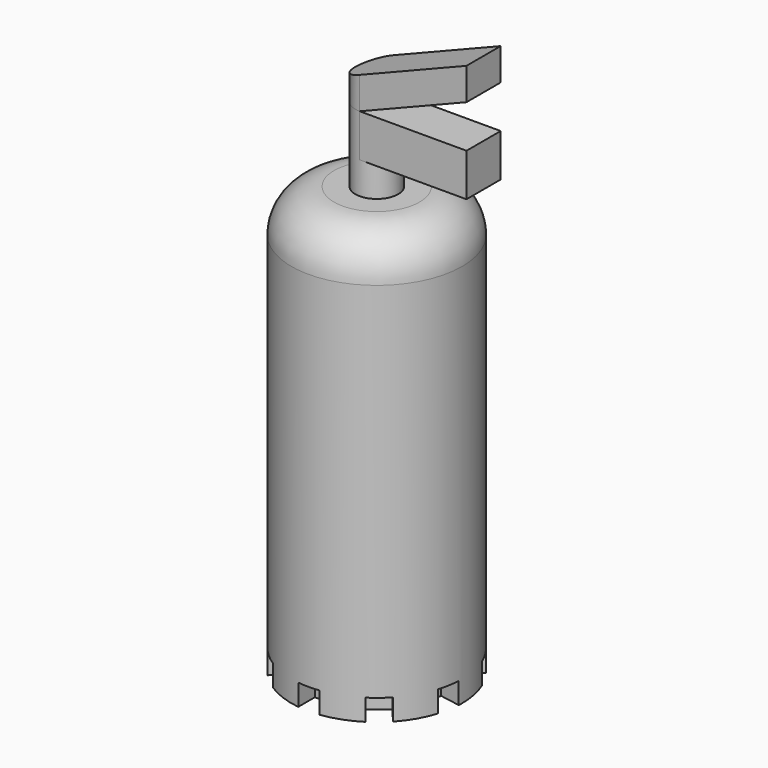
from build123d import *

# Parameters (mm, degrees)
F0_R      = 4
F1_DEPTH  = 20
F2_R      = 2
F3_R      = 1
F4_DEPTH  = 1.5
F6_DEPTH  = 2
F8_DEPTH  = 2
F9_R      = 0.9999
F11_DEPTH = 1


# Not quite as in the source:
# - a fillet or chamfer is up to 0.001 mm smaller than in the source, because OpenCascade refuses the exact size


with BuildPart() as f1:
    # F0 (on Top) → F1 (new body)
    with BuildSketch(Plane.XY):
        Circle(F0_R)
    extrude(amount=F1_DEPTH)

    # F2
    f2_edges = [f1.edges().sort_by_distance(p)[0] for p in [
        (-4, 0, 20),
    ]]
    fillet(f2_edges, radius=F2_R)

    # F3 (on face) → F4 (join)
    with BuildSketch(Plane.XY.offset(20)):
        Circle(F3_R)
    extrude(amount=F4_DEPTH)

    # F5 (on face) → F6 (join)
    with BuildSketch(Plane.XY.offset(21.5)):
        with BuildLine():
            Line((5, 1), (0, 1))
            ThreePointArc((0, 1), (-1, 0), (0, -1))
            Line((0, -1), (5, -1))
            Line((5, -1), (5, 1))
        make_face()
    extrude(amount=F6_DEPTH)

    # F7 (on face) → F8 (join)
    with BuildSketch(Plane.XZ.offset(1)):
        Polygon((-1, 23.5), (0, 23.5), (5, 25.5), (5, 27), (-1, 24.6), align=None)
    extrude(amount=-F8_DEPTH)

    # F9 (radius 1 in the source; OpenCascade refuses exactly that, so slightly less here)
    f9_edges = [f1.edges().sort_by_distance(p)[0] for p in [
        (-1, -1, 24.05),
        (-1, 1, 24.05),
    ]]
    fillet(f9_edges, radius=F9_R)

    # F10 (on face) → F11 (cut)
    with BuildSketch(Plane(origin=(0, 0, 0), x_dir=(1, 0, 0), z_dir=(0, 0, -1))):
        Polygon((0.5, 4), (0, 4), (-0.5, 4), (-0.5, 3), (0.5, 3), align=None)
        Polygon((2.3113850506, 1.9767395245), (2.9541726603, 2.7427839676), (2.5711504387, 3.0641777725), (2.1881282172, 3.3855715773), (1.5453406075, 2.6195271342), align=None)
        Polygon((3.0412473479, 0.0285406565), (4.0260551009, 0.2021888342), (3.939231012, 0.6945927107), (3.8524069232, 1.1869965872), (2.8675991702, 1.0133484095), align=None)
        Polygon((2.3480762114, -1.9330127019), (3.2141016151, -2.4330127019), (3.4641016151, -2), (3.7141016151, -1.5669872981), (2.8480762114, -1.0669872981), align=None)
        Polygon((0.5562141196, -2.990087934), (0.8982342629, -3.9297805548), (1.3680805733, -3.7587704831), (1.8379268837, -3.5877604115), (1.4959067404, -2.6480677907), align=None)
        Polygon((-1.4959067404, -2.6480677907), (-1.8379268837, -3.5877604115), (-1.3680805733, -3.7587704831), (-0.8982342629, -3.9297805548), (-0.5562141196, -2.990087934), align=None)
        Polygon((-2.8480762114, -1.0669872981), (-3.7141016151, -1.5669872981), (-3.4641016151, -2), (-3.2141016151, -2.4330127019), (-2.3480762114, -1.9330127019), align=None)
        Polygon((-2.8675991702, 1.0133484095), (-3.8524069232, 1.1869965872), (-3.939231012, 0.6945927107), (-4.0260551009, 0.2021888342), (-3.0412473479, 0.0285406565), align=None)
        Polygon((-1.5453406075, 2.6195271342), (-2.1881282172, 3.3855715773), (-2.5711504387, 3.0641777725), (-2.9541726603, 2.7427839676), (-2.3113850506, 1.9767395245), align=None)
    extrude(amount=-F11_DEPTH, mode=Mode.SUBTRACT)


solid = f1.part
